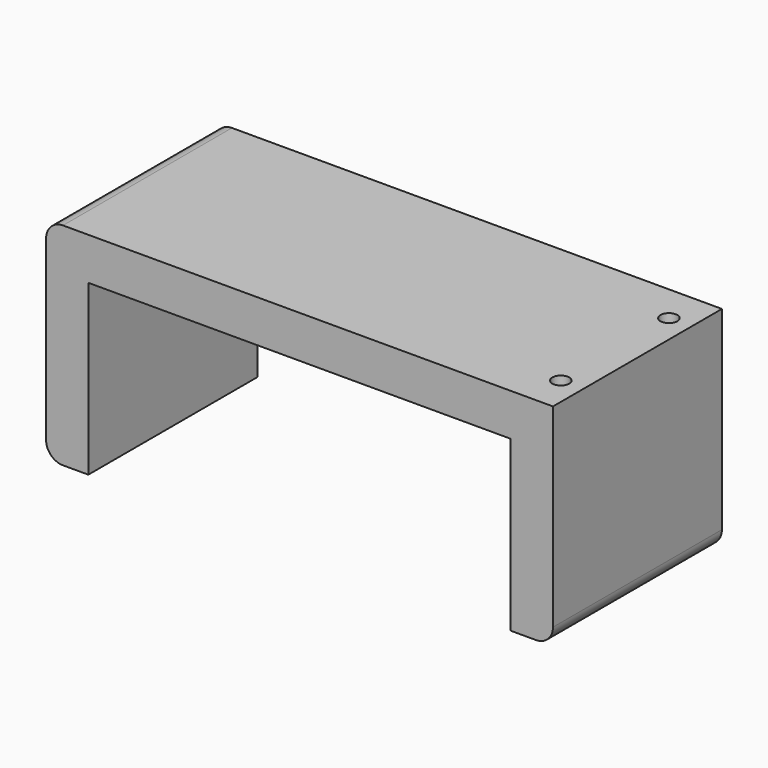
from build123d import *

# Parameters (mm, degrees)
F1_DEPTH = 12.5
F3_R     = 2
F4_D     = 2
F4_DEPTH = 12
F4_TIP   = 0.600860619


# Not quite as in the source:
# - a feature names something its author has since deleted; it is built from what else it names


with BuildPart() as f1:
    # F0 (on Front) → F1 (new body, symmetric)
    with BuildSketch(Plane.XZ):
        Polygon((30.1726347237, 0), (-29.8273652763, 0), (-29.8273652763, -25), (-24.8273652763, -25), (-24.8273652763, -5), (25.1726347237, -5), (25.1726347237, -25), (30.1726347237, -25), align=None)
    extrude(amount=F1_DEPTH, both=True)

    # F3
    f3_edges = [f1.edges().sort_by_distance(p)[0] for p in [
        (30.172635, 0, -25),
        (-29.827365, 0, -25),
        (-29.827365, 0, 0),
    ]]
    fillet(f3_edges, radius=F3_R)

    # F4
    with Locations(Plane.XY):
        with Locations((27.5, 8), (27.5, -8)):
            Hole(F4_D / 2, depth=F4_DEPTH)
            with Locations((0, 0, -(F4_DEPTH + F4_TIP / 2))):  # 118° drill point
                Cone(0, F4_D / 2, F4_TIP, mode=Mode.SUBTRACT)


solid = f1.part
